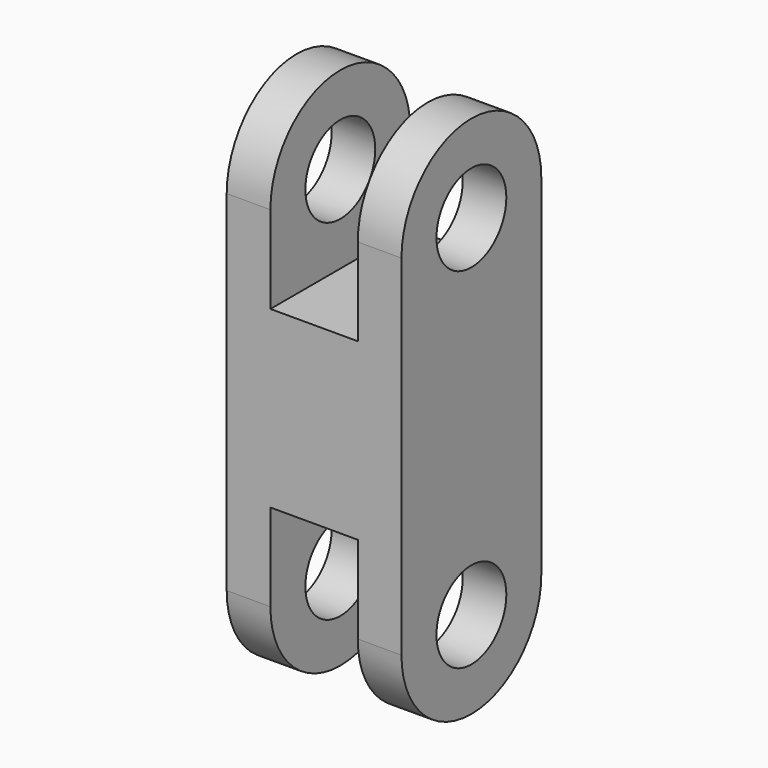
from build123d import *

# Parameters (mm, degrees)
F0_W     = 40
F0_H     = 80
F1_DEPTH = 20
F2_R     = 10
F3_DEPTH = 10
F5_W     = 20
F5_H     = 40
F6_DEPTH = 40
F7_R     = 10
F8_DEPTH = 40
F9_R     = 20
F10_R    = 19.99999


# Not quite as in the source:
# - a fillet or chamfer is up to 0.001 mm smaller than in the source, because OpenCascade refuses the exact size


with BuildPart() as f1:
    # F0 (on Right) → F1 (new body)
    with BuildSketch(Plane.YZ):
        with Locations((20, 40)):
            Rectangle(F0_W, F0_H)
    extrude(amount=F1_DEPTH)

    # F2 (on face) → F3 (join)
    with BuildSketch(Plane.YZ.offset(20)):
        with BuildLine():
            Line((0, 100), (0, 80))
            Line((0, 80), (40, 80))
            Line((40, 80), (40, 100))
            ThreePointArc((40, 100), (20, 120), (0, 100))
        make_face()
        with Locations((20, 100)):
            Circle(F2_R, mode=Mode.SUBTRACT)
    extrude(amount=-F3_DEPTH)

    # F4: F1 across face


with BuildPart() as f1_1:
    add(f1.part)
    add(f1.part.mirror(Plane(origin=(0, 20, 40), x_dir=(0, 1, 0), z_dir=(-1, 0, 0))))

    # F5 (on face) → F6 (cut, through all)
    with BuildSketch(Plane(origin=(0, 40, 0), x_dir=(-1, 0, 0), z_dir=(0, 1, 0))):
        with Locations((0, 20)):
            Rectangle(F5_W, F5_H)
    extrude(amount=-F6_DEPTH, mode=Mode.SUBTRACT)

    # F7 (on face) → F8 (cut, through all)
    with BuildSketch(Plane.YZ.offset(20)):
        with Locations((20, 20)):
            Circle(F7_R)
    extrude(amount=-F8_DEPTH, mode=Mode.SUBTRACT)

    # F9
    f9_edges = [f1_1.edges().sort_by_distance(p)[0] for p in [
        (-15, 0, 0),
    ]]
    fillet(f9_edges, radius=F9_R)

    # F10 (radius 20 in the source; OpenCascade refuses exactly that, so slightly less here)
    f10_edges = [f1_1.edges().sort_by_distance(p)[0] for p in [
        (-15, 40, 0),
        (15, 40, 0),
        (15, 0, 0),
    ]]
    fillet(f10_edges, radius=F10_R)


solid = f1_1.part
